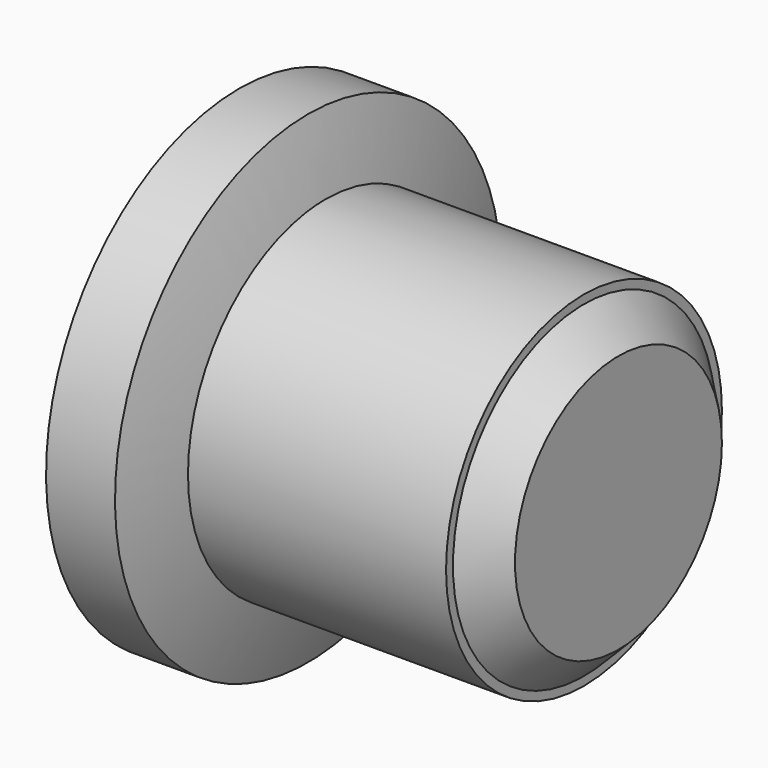
from build123d import *

# Parameters (mm, degrees)
F2_R     = 5
F3_DEPTH = 10
F4_R     = 4.75
F5_DEPTH = 1
F6_SIZE  = 0.99999


# Not quite as in the source:
# - a fillet or chamfer is up to 0.001 mm smaller than in the source, because OpenCascade refuses the exact size


with BuildPart() as f1:
    # F0 (on Front) → F1 (revolve)
    with BuildSketch(Plane.XZ):
        with BuildLine():
            Line((-3.0435194335, 0), (0, 0))
            ThreePointArc((0, 0), (-0.2623133647, 3.5386767586), (-1.0435194335, 7))
            Line((-1.0435194335, 7), (-3.0435194335, 7))
            Line((-3.0435194335, 7), (-3.0435194335, 0))
        make_face()
    revolve(axis=Axis((-1.5217597168, 0, 0), (1, 0, 0)))

    # F2 (on face) → F3 (join)
    with BuildSketch(Plane(origin=(-3.0435194335, 0, 0), x_dir=(0, -1, 0), z_dir=(-1, 0, 0))):
        Circle(F2_R)
    extrude(amount=-F3_DEPTH)

    # F4 (on face) → F5 (join)
    with BuildSketch(Plane.YZ.offset(6.9564805665)):
        Circle(F4_R)
    extrude(amount=F5_DEPTH)

    # F6 (size 1 in the source; OpenCascade refuses exactly that, so slightly less here)
    f6_edges = [f1.edges().sort_by_distance(p)[0] for p in [
        (7.956481, -4.75, 0),
    ]]
    chamfer(f6_edges, length=F6_SIZE)


solid = f1.part
